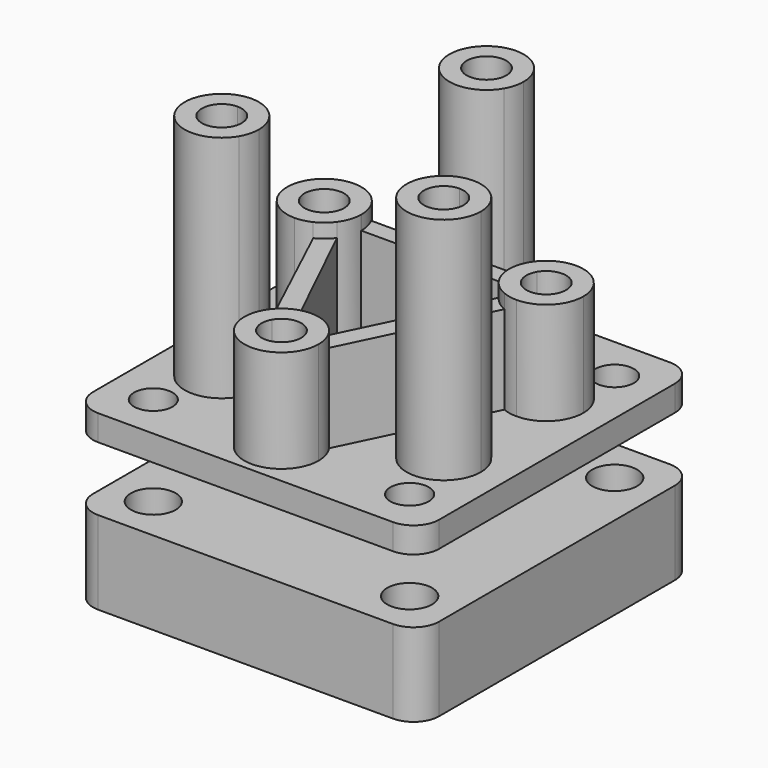
from build123d import *

# Parameters (mm, degrees)
F0_W      = 27
F0_H      = 27
F1_DEPTH  = 2
F2_R      = 1.5
F3_DEPTH  = 5
F4_R      = 2
F7_DEPTH  = 17.9
F8_DEPTH  = 8
F9_DEPTH  = 2
F11_DEPTH = 6.9
F13_R     = 1.75
F14_DEPTH = 6.5


# Not quite as in the source:
# - the program builds the solid bodies; features that only make, move or delete a surface that nothing else refers to are left out


with BuildPart() as f1:
    # F0 (on Top) → F1 (new body)
    with BuildSketch(Plane.XY):
        Rectangle(F0_W, F0_H)
    extrude(amount=F1_DEPTH)

    # F2 (on face) → F3 (cut)
    with BuildSketch(Plane.XY.offset(2)):
        with Locations((-10, 10)):
            Circle(F2_R)
        with Locations((10, 10)):
            Circle(F2_R)
        with Locations((10, -10)):
            Circle(F2_R)
        with Locations((-10, -10)):
            Circle(F2_R)
    extrude(amount=-F3_DEPTH, mode=Mode.SUBTRACT)

    # F4
    f4_edges = [f1.edges().sort_by_distance(p)[0] for p in [
        (13.5, -13.5, 1),
        (-13.5, 13.5, 1),
        (13.5, 13.5, 1),
        (-13.5, -13.5, 1),
    ]]
    fillet(f4_edges, radius=F4_R)

    # F6 (on face) → F9 (cut)
    with BuildSketch(Plane.XY.offset(2)):
        with BuildLine():
            Line((8.6602540378, -5), (7.317914662, -5.775))
            ThreePointArc((7.317914662, -5.775), (9.0614235578, -6.4971850307), (10.2102540378, -5))
            ThreePointArc((10.2102540378, -5), (9.7562695487, -3.9039844892), (8.6602540378, -3.45))
            Line((8.6602540378, -3.45), (8.6602540378, -5))
        make_face()
        with BuildLine():
            ThreePointArc((8.6602540378, -3.45), (7.317914662, -4.225), (7.317914662, -5.775))
            Line((7.317914662, -5.775), (8.6602540378, -5))
            Line((8.6602540378, -5), (8.6602540378, -3.45))
        make_face()
        with BuildLine():
            ThreePointArc((1.55, 10), (-0.4011695199, 11.4971850307), (-1.3423393759, 9.225))
            Line((-1.3423393759, 9.225), (0, 10))
            Line((0, 10), (1.3423393759, 9.225))
            ThreePointArc((1.3423393759, 9.225), (1.4971850307, 9.5988304801), (1.55, 10))
        make_face()
        with BuildLine():
            Line((0, 10), (-1.3423393759, 9.225))
            ThreePointArc((-1.3423393759, 9.225), (0, 8.45), (1.3423393759, 9.225))
            Line((1.3423393759, 9.225), (0, 10))
        make_face()
        with BuildLine():
            ThreePointArc((7.317914662, 5.775), (7.317914662, 4.225), (8.6602540378, 3.45))
            Line((8.6602540378, 3.45), (8.6602540378, 5))
            Line((8.6602540378, 5), (7.317914662, 5.775))
        make_face()
        with BuildLine():
            Line((8.6602540378, 5), (8.6602540378, 3.45))
            ThreePointArc((8.6602540378, 3.45), (9.7562695487, 3.9039844892), (10.2102540378, 5))
            ThreePointArc((10.2102540378, 5), (9.0614235578, 6.4971850307), (7.317914662, 5.775))
            Line((7.317914662, 5.775), (8.6602540378, 5))
        make_face()
        with BuildLine():
            ThreePointArc((-7.317914662, 5.775), (-10.0025934137, 5.775), (-8.6602540378, 3.45))
            Line((-8.6602540378, 3.45), (-8.6602540378, 5))
            Line((-8.6602540378, 5), (-7.317914662, 5.775))
        make_face()
        with BuildLine():
            Line((-8.6602540378, 5), (-8.6602540378, 3.45))
            ThreePointArc((-8.6602540378, 3.45), (-7.564238527, 3.9039844892), (-7.1102540378, 5))
            ThreePointArc((-7.1102540378, 5), (-7.1630690071, 5.4011695199), (-7.317914662, 5.775))
            Line((-7.317914662, 5.775), (-8.6602540378, 5))
        make_face()
        with BuildLine():
            ThreePointArc((-8.6602540378, -3.45), (-10.0025934137, -5.775), (-7.317914662, -5.775))
            Line((-7.317914662, -5.775), (-8.6602540378, -5))
            Line((-8.6602540378, -5), (-8.6602540378, -3.45))
        make_face()
        with BuildLine():
            Line((-8.6602540378, -5), (-7.317914662, -5.775))
            ThreePointArc((-7.317914662, -5.775), (-7.1630690071, -5.4011695199), (-7.1102540378, -5))
            ThreePointArc((-7.1102540378, -5), (-7.564238527, -3.9039844892), (-8.6602540378, -3.45))
            Line((-8.6602540378, -3.45), (-8.6602540378, -5))
        make_face()
        with BuildLine():
            Line((-1.3423393759, -9.225), (0, -10))
            Line((0, -10), (1.3423393759, -9.225))
            ThreePointArc((1.3423393759, -9.225), (0, -8.45), (-1.3423393759, -9.225))
        make_face()
        with BuildLine():
            Line((1.3423393759, -9.225), (0, -10))
            Line((0, -10), (-1.3423393759, -9.225))
            ThreePointArc((-1.3423393759, -9.225), (-0.4011695199, -11.4971850307), (1.55, -10))
            ThreePointArc((1.55, -10), (1.4971850307, -9.5988304801), (1.3423393759, -9.225))
        make_face()
    extrude(amount=-F9_DEPTH, mode=Mode.SUBTRACT)


with BuildPart() as f7:
    # F6 (on face) → F7 (new body)
    with BuildSketch(Plane.XY.offset(2)):
        with BuildLine():
            ThreePointArc((2.9, 10), (-0.7505752308, 12.8011848962), (-2.511473671, 8.55))
            Line((-2.511473671, 8.55), (-1.3423393759, 9.225))
            ThreePointArc((-1.3423393759, 9.225), (-0.4011695199, 11.4971850307), (1.55, 10))
            ThreePointArc((1.55, 10), (1.4971850307, 9.5988304801), (1.3423393759, 9.225))
            Line((1.3423393759, 9.225), (2.511473671, 8.55))
            ThreePointArc((2.511473671, 8.55), (2.8011848962, 9.2494247692), (2.9, 10))
        make_face()
        with BuildLine():
            Line((-1.3423393759, 9.225), (-2.511473671, 8.55))
            ThreePointArc((-2.511473671, 8.55), (0, 7.1), (2.511473671, 8.55))
            Line((2.511473671, 8.55), (1.3423393759, 9.225))
            ThreePointArc((1.3423393759, 9.225), (0, 8.45), (-1.3423393759, 9.225))
        make_face()
    extrude(amount=F7_DEPTH)


with BuildPart() as f7b:
    # F6 (on face) → F7, piece 2 (new body)
    with BuildSketch(Plane.XY.offset(2)):
        with BuildLine():
            Line((7.317914662, -5.775), (6.1487803669, -6.45))
            ThreePointArc((6.1487803669, -6.45), (9.4108292686, -7.8011848962), (11.5602540378, -5))
            ThreePointArc((11.5602540378, -5), (10.7108637033, -2.9493903346), (8.6602540378, -2.1))
            Line((8.6602540378, -2.1), (8.6602540378, -3.45))
            ThreePointArc((8.6602540378, -3.45), (9.7562695487, -3.9039844892), (10.2102540378, -5))
            ThreePointArc((10.2102540378, -5), (9.0614235578, -6.4971850307), (7.317914662, -5.775))
        make_face()
        with BuildLine():
            ThreePointArc((8.6602540378, -2.1), (6.1487803669, -3.55), (6.1487803669, -6.45))
            Line((6.1487803669, -6.45), (7.317914662, -5.775))
            ThreePointArc((7.317914662, -5.775), (7.317914662, -4.225), (8.6602540378, -3.45))
            Line((8.6602540378, -3.45), (8.6602540378, -2.1))
        make_face()
    extrude(amount=F7_DEPTH)


with BuildPart() as f7c:
    # F6 (on face) → F7, piece 3 (new body)
    with BuildSketch(Plane.XY.offset(2)):
        with BuildLine():
            ThreePointArc((-8.6602540378, -2.1), (-11.1717277088, -6.45), (-6.1487803669, -6.45))
            Line((-6.1487803669, -6.45), (-7.317914662, -5.775))
            ThreePointArc((-7.317914662, -5.775), (-10.0025934137, -5.775), (-8.6602540378, -3.45))
            Line((-8.6602540378, -3.45), (-8.6602540378, -2.1))
        make_face()
        with BuildLine():
            Line((-7.317914662, -5.775), (-6.1487803669, -6.45))
            ThreePointArc((-6.1487803669, -6.45), (-5.8590691416, -5.7505752308), (-5.7602540378, -5))
            ThreePointArc((-5.7602540378, -5), (-6.6096443724, -2.9493903346), (-8.6602540378, -2.1))
            Line((-8.6602540378, -2.1), (-8.6602540378, -3.45))
            ThreePointArc((-8.6602540378, -3.45), (-7.564238527, -3.9039844892), (-7.1102540378, -5))
            ThreePointArc((-7.1102540378, -5), (-7.1630690071, -5.4011695199), (-7.317914662, -5.775))
        make_face()
    extrude(amount=F7_DEPTH)


with BuildPart() as f8:
    # F6 (on face) → F8 (new body)
    with BuildSketch(Plane.XY.offset(2)):
        with BuildLine():
            ThreePointArc((-6.1487803669, 6.45), (-11.1717277088, 6.45), (-8.6602540378, 2.1))
            Line((-8.6602540378, 2.1), (-8.6602540378, 3.45))
            ThreePointArc((-8.6602540378, 3.45), (-10.0025934137, 5.775), (-7.317914662, 5.775))
            Line((-7.317914662, 5.775), (-6.1487803669, 6.45))
        make_face()
        with BuildLine():
            Line((-8.6602540378, 3.45), (-8.6602540378, 2.1))
            ThreePointArc((-8.6602540378, 2.1), (-8.0292332503, 2.1694854239), (-7.4284515985, 2.3746118857))
            ThreePointArc((-7.4284515985, 2.3746118857), (-6.8099472018, 2.7669830694), (-6.3094802441, 3.3018060856))
            ThreePointArc((-6.3094802441, 3.3018060856), (-5.9042419792, 4.0975602331), (-5.7603309126, 4.9788844183))
            ThreePointArc((-5.7603309126, 4.9788844183), (-5.7602732566, 4.9894421392), (-5.7602540378, 5))
            ThreePointArc((-5.7602540378, 5), (-5.8488031659, 5.7111568004), (-6.1090429997, 6.3788844183))
            ThreePointArc((-6.1090429997, 6.3788844183), (-6.1286619553, 6.4145817501), (-6.1487803669, 6.45))
            Line((-6.1487803669, 6.45), (-7.317914662, 5.775))
            ThreePointArc((-7.317914662, 5.775), (-7.1630690071, 5.4011695199), (-7.1102540378, 5))
            ThreePointArc((-7.1102540378, 5), (-7.564238527, 3.9039844892), (-8.6602540378, 3.45))
        make_face()
    extrude(amount=F8_DEPTH)


with BuildPart() as f8b:
    # F6 (on face) → F8, piece 2 (new body)
    with BuildSketch(Plane.XY.offset(2)):
        with BuildLine():
            ThreePointArc((6.3094802441, 3.3018060856), (6.8540944049, 2.7311264072), (7.5323514668, 2.3283271551))
            ThreePointArc((7.5323514668, 2.3283271551), (8.0848634098, 2.1576549075), (8.6602540378, 2.1))
            Line((8.6602540378, 2.1), (8.6602540378, 3.45))
            ThreePointArc((8.6602540378, 3.45), (7.317914662, 4.225), (7.317914662, 5.775))
            Line((7.317914662, 5.775), (6.1487803669, 6.45))
            ThreePointArc((6.1487803669, 6.45), (6.1286619553, 6.4145817501), (6.1090429997, 6.3788844183))
            ThreePointArc((6.1090429997, 6.3788844183), (5.8462327308, 5.7009166023), (5.7603309126, 4.9788844183))
            ThreePointArc((5.7603309126, 4.9788844183), (5.9042419792, 4.0975602331), (6.3094802441, 3.3018060856))
        make_face()
        with BuildLine():
            Line((8.6602540378, 3.45), (8.6602540378, 2.1))
            ThreePointArc((8.6602540378, 2.1), (10.7108637033, 2.9493903346), (11.5602540378, 5))
            ThreePointArc((11.5602540378, 5), (9.4108292686, 7.8011848962), (6.1487803669, 6.45))
            Line((6.1487803669, 6.45), (7.317914662, 5.775))
            ThreePointArc((7.317914662, 5.775), (9.0614235578, 6.4971850307), (10.2102540378, 5))
            ThreePointArc((10.2102540378, 5), (9.7562695487, 3.9039844892), (8.6602540378, 3.45))
        make_face()
    extrude(amount=F8_DEPTH)


with BuildPart() as f8c:
    # F6 (on face) → F8, piece 3 (new body)
    with BuildSketch(Plane.XY.offset(2)):
        with BuildLine():
            ThreePointArc((1.55, -10), (-0.4011695199, -11.4971850307), (-1.3423393759, -9.225))
            Line((-1.3423393759, -9.225), (-2.511473671, -8.55))
            ThreePointArc((-2.511473671, -8.55), (-0.7505752308, -12.8011848962), (2.9, -10))
            ThreePointArc((2.9, -10), (2.8011848962, -9.2494247692), (2.511473671, -8.55))
            Line((2.511473671, -8.55), (1.3423393759, -9.225))
            ThreePointArc((1.3423393759, -9.225), (1.4971850307, -9.5988304801), (1.55, -10))
        make_face()
        with BuildLine():
            Line((-2.511473671, -8.55), (-1.3423393759, -9.225))
            ThreePointArc((-1.3423393759, -9.225), (0, -8.45), (1.3423393759, -9.225))
            Line((1.3423393759, -9.225), (2.511473671, -8.55))
            ThreePointArc((2.511473671, -8.55), (2.4434921556, -8.4381593918), (2.3705336425, -8.3295))
            ThreePointArc((2.3705336425, -8.3295), (1.8310495376, -7.7511652816), (1.1553766827, -7.3400930992))
            ThreePointArc((1.1553766827, -7.3400930992), (0, -7.1), (-1.1553766827, -7.3400930992))
            ThreePointArc((-1.1553766827, -7.3400930992), (-1.8408719481, -7.759198699), (-2.3850615189, -8.3503086497))
            ThreePointArc((-2.3850615189, -8.3503086497), (-2.4503027109, -8.4488660197), (-2.511473671, -8.55))
        make_face()
    extrude(amount=F8_DEPTH)


with BuildPart() as f11:
    # F6 (on face) → F11 (new body)
    with BuildSketch(Plane.XY.offset(2)):
        with BuildLine():
            Line((-7.1770187587, 1.855467693), (-2.3850615189, -8.3503086497))
            ThreePointArc((-2.3850615189, -8.3503086497), (-1.8408719481, -7.759198699), (-1.1553766827, -7.3400930992))
            Line((-1.1553766827, -7.3400930992), (-6.3094802441, 3.3018060856))
            ThreePointArc((-6.3094802441, 3.3018060856), (-6.8099472018, 2.7669830694), (-7.4284515985, 2.3746118857))
            Line((-7.4284515985, 2.3746118857), (-7.1770187587, 1.855467693))
        make_face()
    extrude(amount=F11_DEPTH)


with BuildPart() as f11b:
    # F6 (on face) → F11, piece 2 (new body)
    with BuildSketch(Plane.XY.offset(2)):
        with BuildLine():
            ThreePointArc((-5.7602540378, 5), (-5.7602732566, 4.9894421392), (-5.7603309126, 4.9788844183))
            Line((-5.7603309126, 4.9788844183), (5.7603309126, 4.9788844183))
            ThreePointArc((5.7603309126, 4.9788844183), (5.8462327308, 5.7009166023), (6.1090429997, 6.3788844183))
            Line((6.1090429997, 6.3788844183), (0, 6.3788844183))
            Line((0, 6.3788844183), (-6.1090429997, 6.3788844183))
            ThreePointArc((-6.1090429997, 6.3788844183), (-5.8488031659, 5.7111568004), (-5.7602540378, 5))
        make_face()
    extrude(amount=F11_DEPTH)


with BuildPart() as f11c:
    # F6 (on face) → F11, piece 3 (new body)
    with BuildSketch(Plane.XY.offset(2)):
        with BuildLine():
            ThreePointArc((1.1553766827, -7.3400930992), (1.8310495376, -7.7511652816), (2.3705336425, -8.3295))
            Line((2.3705336425, -8.3295), (7.5323514668, 2.3283271551))
            ThreePointArc((7.5323514668, 2.3283271551), (6.8540944049, 2.7311264072), (6.3094802441, 3.3018060856))
            Line((6.3094802441, 3.3018060856), (1.1553766827, -7.3400930992))
        make_face()
    extrude(amount=F11_DEPTH)


with BuildPart() as f14:
    # F13 (on offset) → F14 (new body)
    with BuildSketch(Plane.XY.offset(-5)):
        with BuildLine():
            Line((-11.5, -13.5), (11.5, -13.5))
            ThreePointArc((11.5, -13.5), (12.9142135624, -12.9142135624), (13.5, -11.5))
            Line((13.5, -11.5), (13.5, 11.5))
            ThreePointArc((13.5, 11.5), (12.9142135624, 12.9142135624), (11.5, 13.5))
            Line((11.5, 13.5), (-11.5, 13.5))
            ThreePointArc((-11.5, 13.5), (-12.9142135624, 12.9142135624), (-13.5, 11.5))
            Line((-13.5, 11.5), (-13.5, -11.5))
            ThreePointArc((-13.5, -11.5), (-12.9142135624, -12.9142135624), (-11.5, -13.5))
        make_face()
        with Locations((-10, -10)):
            Circle(F13_R, mode=Mode.SUBTRACT)
        with Locations((10, -10)):
            Circle(F13_R, mode=Mode.SUBTRACT)
        with Locations((-10, 10)):
            Circle(F13_R, mode=Mode.SUBTRACT)
        with Locations((10, 10)):
            Circle(F13_R, mode=Mode.SUBTRACT)
    extrude(amount=-F14_DEPTH)


solid = Compound([f1.part, f7.part, f7b.part, f7c.part, f8.part, f8b.part, f8c.part, f11.part, f11b.part, f11c.part, f14.part])
